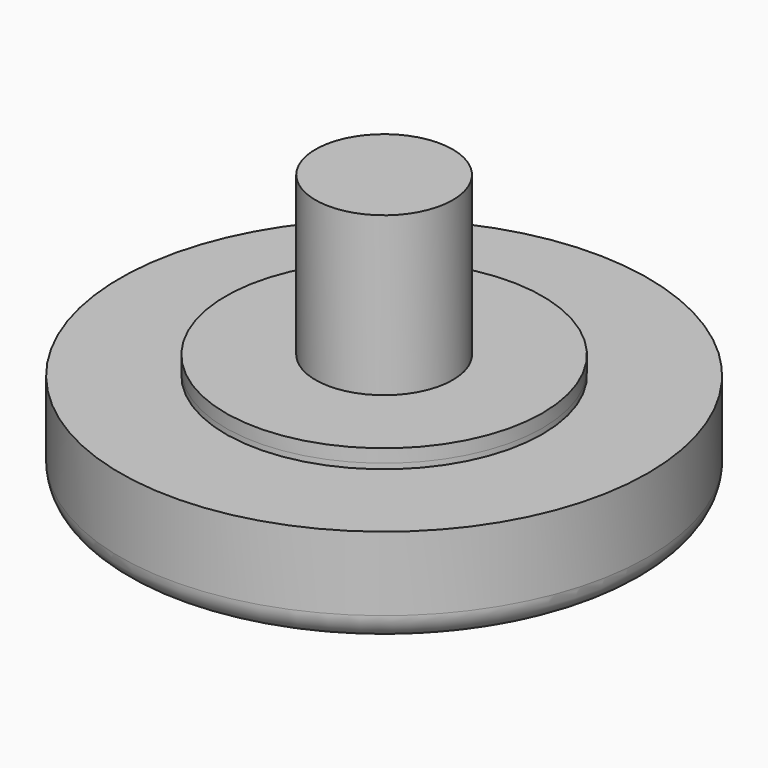
from build123d import *

# Parameters (mm, degrees)
F0_R     = 10
F0_R_2   = 6
F1_DEPTH = 4
F0_R_3   = 2.6
F2_DEPTH = 4.5
F3_DEPTH = 10.5
F4_R     = 8.5
F5_DEPTH = 1.5
F7_R     = 1
F8_DEPTH = 0.2


# Not quite as in the source:
# - a fillet or chamfer that OpenCascade refuses, or shapes differently, is made with other operations: its cross-section is extruded or revolved along the edge and cut away or added


with BuildPart() as f1:
    # F0 (on Top) → F1 (new body)
    with BuildSketch(Plane.XY):
        with Locations((-11.3181825727, 20.5227266997)):
            Circle(F0_R)
        with Locations((-11.3181825727, 20.5227266997)):
            Circle(F0_R_2, mode=Mode.SUBTRACT)
    extrude(amount=F1_DEPTH)

    # F0 (on Top) → F2 (join)
    with BuildSketch(Plane.XY):
        with Locations((-11.3181825727, 20.5227266997)):
            Circle(F0_R_2)
        with Locations((-11.3181825727, 20.5227266997)):
            Circle(F0_R_3, mode=Mode.SUBTRACT)
    extrude(amount=F2_DEPTH)

    # F0 (on Top) → F3 (join)
    with BuildSketch(Plane.XY):
        with Locations((-11.3181825727, 20.5227266997)):
            Circle(F0_R_3)
    extrude(amount=F3_DEPTH)

    # F4 (on face) → F5 (cut)
    with BuildSketch(Plane(origin=(0, 0, 0), x_dir=(1, 0, 0), z_dir=(0, 0, -1))):
        with Locations((-11.3181825727, -20.5227266997)):
            Circle(F4_R)
    extrude(amount=-F5_DEPTH, mode=Mode.SUBTRACT)

    # F6: fillet of radius 20 on 1 edges, made by hand

    # F6_s1 → F6_t2 (revolve)
    with BuildSketch(Plane.XZ.offset(-20.5227266997)):
        with BuildLine():
            ThreePointArc((-2.8181825727, 0), (-6.5445413033, 1.1214168703), (-10.4175246495, 1.5))
            Line((-10.4175246495, 1.5), (-2.8181825727, 1.5))
            Line((-2.8181825727, 1.5), (-2.8181825727, 0))
        make_face()
    revolve(axis=Axis((-11.3181825727, 20.5227266997, 1.5), (0, 0, -1)))

    # F7
    f7_edges = [f1.edges().sort_by_distance(p)[0] for p in [
        (-21.318183, 20.522727, 0),
    ]]
    fillet(f7_edges, radius=F7_R)

    # F8 (cut): a face of the model
    f8_faces = [f1.faces().sort_by_distance(p)[0] for p in [
        (-21.0353398602, 20.5227266997, 4),
    ]]
    extrude(f8_faces, amount=-F8_DEPTH, mode=Mode.SUBTRACT)


solid = f1.part
